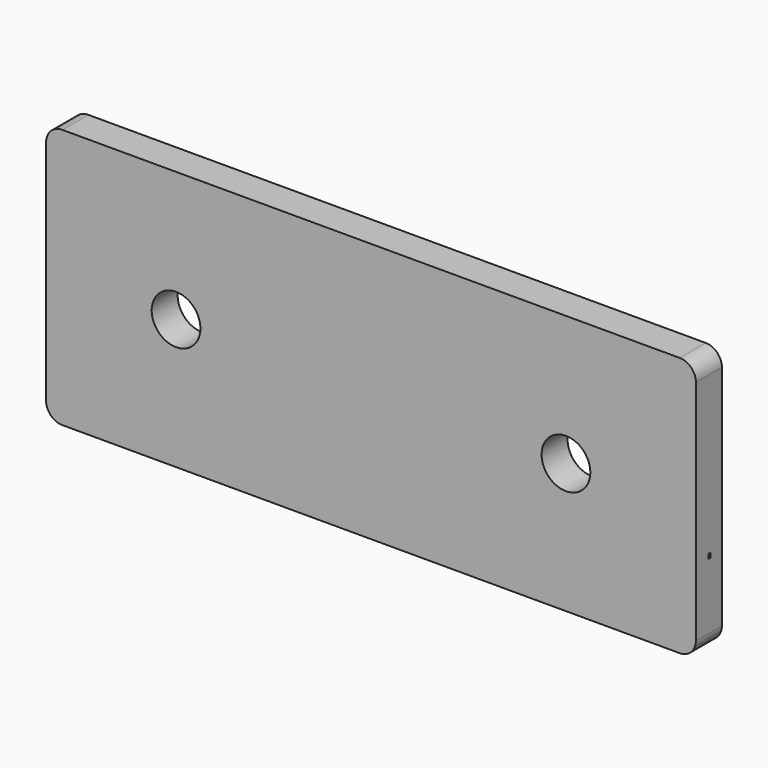
from build123d import *

# Parameters (mm, degrees)
F0_W     = 254
F0_H     = 101.6
F0_R     = 9.525
F1_DEPTH = 12.7
F2_R     = 6.35
F3_DEPTH = 12.7
F4_R     = 6.35
F5_W     = 0.9328643791
F5_H     = 1.7582587898
F5_W_2   = 0.0005662441
F5_H_2   = 0.0007078052
F6_DEPTH = 254.001


# Not quite as in the source:
# - a feature of the source that left no trace in its solid (it failed there, or was rolled back) is left out


with BuildPart() as f1:
    # F0 (on Front) → F1 (new body)
    with BuildSketch(Plane.XZ):
        with Locations((143.2877514958, 67.8497503132)):
            Rectangle(F0_W, F0_H)
        with Locations((67.0877514958, 67.8497503132)):
            Circle(F0_R, mode=Mode.SUBTRACT)
        with Locations((219.4877514958, 67.8497503132)):
            Circle(F0_R, mode=Mode.SUBTRACT)
    extrude(amount=F1_DEPTH)

    # F2
    f2_edges = [f1.edges().sort_by_distance(p)[0] for p in [
        (16.287751, -6.35, 118.64975),
        (16.287751, -6.35, 17.04975),
        (270.287751, -6.35, 118.64975),
        (270.287751, -6.35, 17.04975),
    ]]
    fillet(f2_edges, radius=F2_R)

    # F0 (on Front) → F3 (join)
    with BuildSketch(Plane.XZ):
        with Locations((143.2877514958, 67.8497503132)):
            Rectangle(F0_W, F0_H)
        with Locations((67.0877514958, 67.8497503132)):
            Circle(F0_R, mode=Mode.SUBTRACT)
        with Locations((219.4877514958, 67.8497503132)):
            Circle(F0_R, mode=Mode.SUBTRACT)
    extrude(amount=F3_DEPTH)

    # F4
    f4_edges = [f1.edges().sort_by_distance(p)[0] for p in [
        (270.287751, -6.35, 118.64975),
        (16.287751, -6.35, 118.64975),
        (270.287751, -6.35, 17.04975),
        (16.287751, -6.35, 17.04975),
    ]]
    fillet(f4_edges, radius=F4_R)

    # F5 (on face) → F6 (cut, through all)
    with BuildSketch(Plane(origin=(16.2877514958, 0, 0), x_dir=(0, -1, 0), z_dir=(-1, 0, 0))):
        with Locations((6.063854089, 49.9223377556)):
            Rectangle(F5_W, F5_H)
        with Locations((8.4549216554, 49.0087680519)):
            Rectangle(F5_W_2, F5_H_2)
    extrude(amount=-F6_DEPTH, mode=Mode.SUBTRACT)


solid = f1.part
